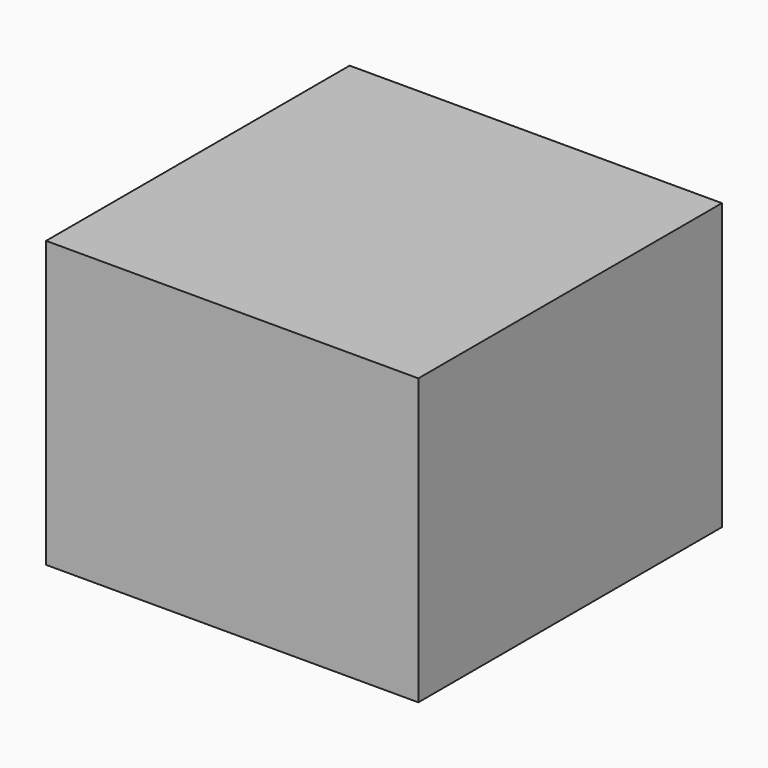
from build123d import *

# Parameters (mm, degrees)
F0_W     = 99.6783301234
F0_H     = 76.3818621635
F1_DEPTH = 101.6


# Not quite as in the source:
# - the program builds the solid bodies; features that only make, move or delete a surface that nothing else refers to are left out


with BuildPart() as f1:
    # F0 (on Front) → F1 (new body)
    with BuildSketch(Plane.XZ):
        with Locations((-49.8391650617, 38.1909310818)):
            Rectangle(F0_W, F0_H)
    extrude(amount=F1_DEPTH)


solid = f1.part
